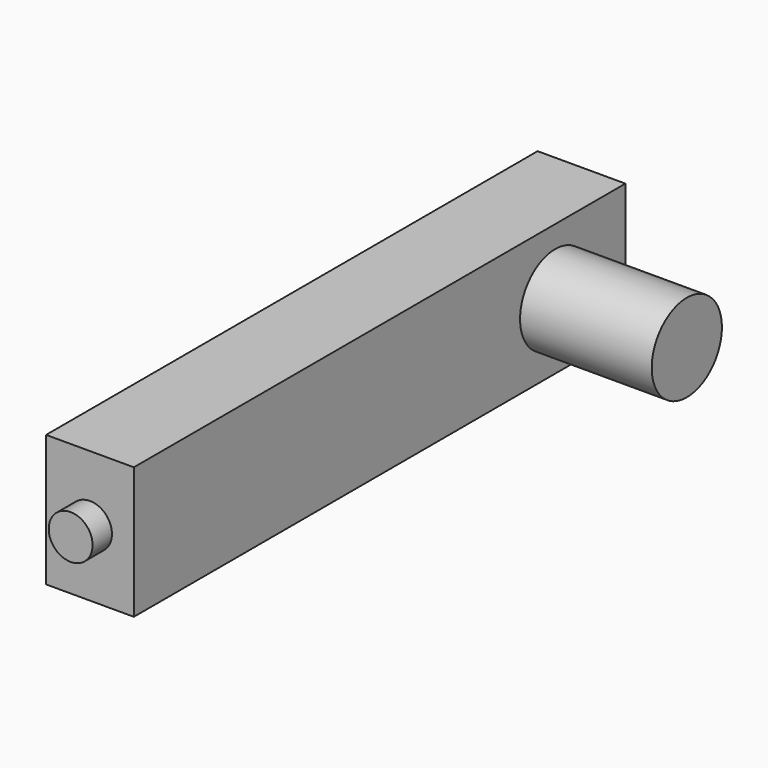
from build123d import *

# Parameters (mm, degrees)
F0_W     = 4
F0_H     = 6
F1_DEPTH = 28
F2_R     = 2
F3_DEPTH = 6
F4_R     = 1
F5_DEPTH = 1.1


# Not quite as in the source:
# - a feature names something its author has since deleted; it is built from what else it names


with BuildPart() as f1:
    # F0 (on Front) → F1 (new body)
    with BuildSketch(Plane.XZ):
        Rectangle(F0_W, F0_H)
    extrude(amount=F1_DEPTH)

    # F2 (on face) → F3 (join)
    with BuildSketch(Plane.YZ.offset(2)):
        with Locations((-4, 0)):
            Circle(F2_R)
    extrude(amount=F3_DEPTH)

    # F4 (on face) → F5 (join)
    with BuildSketch(Plane.XZ.offset(28)):
        Circle(F4_R)
    extrude(amount=F5_DEPTH)


solid = f1.part
